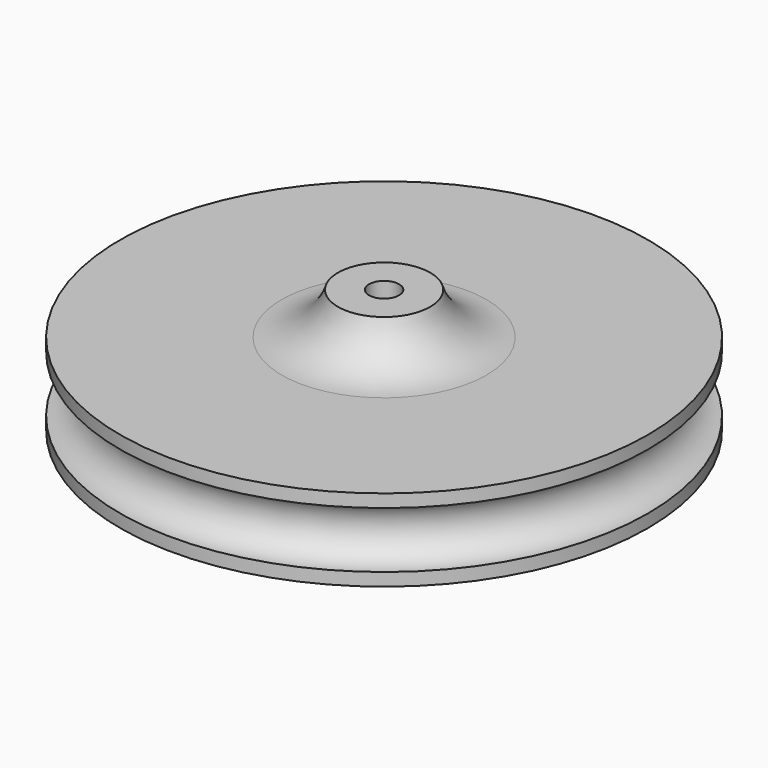
from build123d import *


# Not quite as in the source:
# - a fillet or chamfer that OpenCascade refuses, or shapes differently, is made with other operations: its cross-section is extruded or revolved along the edge and cut away or added


with BuildPart() as f1:
    # F0 (on Front) → F1 (revolve)
    with BuildSketch(Plane.XZ):
        with BuildLine():
            Line((0, 3.2086027786), (0, 0))
            Line((0, 0), (22.5, 0))
            Line((22.5, 0), (22.5, 1.1))
            ThreePointArc((22.5, 1.1), (20.1, 3.5), (22.5, 5.9))
            Line((22.5, 5.9), (22.5, 7))
            Line((22.5, 7), (3.9362940006, 7))
            Line((3.9362940006, 7), (3.9362940006, 10.5700949207))
            Line((3.9362940006, 10.5700949207), (1.281605335, 10.5700949207))
            Line((1.281605335, 10.5700949207), (1.281605335, 3.2086027786))
            Line((1.281605335, 3.2086027786), (0, 3.2086027786))
        make_face()
    revolve(axis=Axis((0, 0, 5.2850474603), (0, 0, -1)))

    # F2: fillet of radius 5 on 1 edges, made by hand

    # F2_s1 → F2_t2 (revolve)
    with BuildSketch(Plane.XZ):
        with BuildLine():
            ThreePointArc((8.7274704182, 7), (5.739956853, 7.9906655542), (3.9362940006, 10.5700949207))
            Line((3.9362940006, 10.5700949207), (3.9362940006, 7))
            Line((3.9362940006, 7), (8.7274704182, 7))
        make_face()
    revolve(axis=Axis((0, 0, 7), (0, 0, -1)))


solid = f1.part
